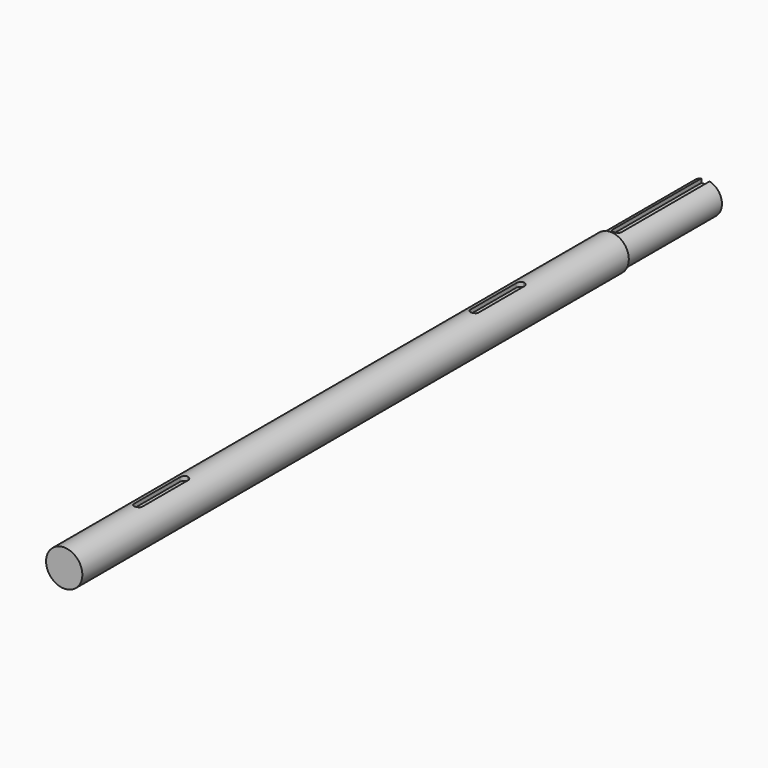
from build123d import *

# Parameters (mm, degrees)
F0_R      = 56.35625
F1_DEPTH  = 2120.9
F2_R      = 50.8
F3_DEPTH  = 368.3
F4_R      = 11.1125
F5_DEPTH  = 34.925
F6_W      = 25.4
F6_H      = 25.4
F7_DEPTH  = 355.6
F8_R      = 12.699
F11_DEPTH = 13.97


# Not quite as in the source:
# - a fillet or chamfer is up to 0.001 mm smaller than in the source, because OpenCascade refuses the exact size


with BuildPart() as f1:
    # F0 (on Front) → F1 (new body)
    with BuildSketch(Plane.XZ):
        Circle(F0_R)
    extrude(amount=-F1_DEPTH)

    # F2 (on face) → F3 (join)
    with BuildSketch(Plane(origin=(0, 2120.9, 0), x_dir=(-1, 0, 0), z_dir=(0, 1, 0))):
        Circle(F2_R)
    extrude(amount=F3_DEPTH)

    # F4 (on face) → F5 (cut)
    with BuildSketch(Plane(origin=(0, 2489.2, 0), x_dir=(-1, 0, 0), z_dir=(0, 1, 0))):
        Circle(F4_R)
    extrude(amount=-F5_DEPTH, mode=Mode.SUBTRACT)

    # F6 (on face) → F7 (cut)
    with BuildSketch(Plane(origin=(0, 2489.2, 0), x_dir=(-1, 0, 0), z_dir=(0, 1, 0))):
        with Locations((0, 49.53)):
            Rectangle(F6_W, F6_H)
    extrude(amount=-F7_DEPTH, mode=Mode.SUBTRACT)

    # F8 (radius 12.7 in the source; OpenCascade refuses exactly that, so slightly less here)
    f8_edges = [f1.edges().sort_by_distance(p)[0] for p in [
        (12.7, 2133.6, 43.008444),
        (-12.7, 2133.6, 43.008444),
    ]]
    fillet(f8_edges, radius=F8_R)

    # F10 (on offset) → F11 (cut)
    with BuildSketch(Plane.XY.offset(56.35625)):
        with BuildLine():
            ThreePointArc((0, 477.8375), (-8.9802561211, 474.1177561211), (-12.7, 465.1375))
            Line((-12.7, 465.1375), (-12.7, 287.3375))
            ThreePointArc((-12.7, 287.3375), (-8.9802561211, 278.3572438789), (0, 274.6375))
            ThreePointArc((0, 274.6375), (8.9802561211, 278.3572438789), (12.7, 287.3375))
            Line((12.7, 287.3375), (12.7, 465.1375))
            ThreePointArc((12.7, 465.1375), (8.9802561211, 474.1177561211), (0, 477.8375))
        make_face()
        with BuildLine():
            ThreePointArc((0, 1782.7625), (-8.9802561211, 1779.0427561211), (-12.7, 1770.0625))
            Line((-12.7, 1770.0625), (-12.7, 1592.2625))
            ThreePointArc((-12.7, 1592.2625), (-8.9802561211, 1583.2822438789), (0, 1579.5625))
            ThreePointArc((0, 1579.5625), (8.9802561211, 1583.2822438789), (12.7, 1592.2625))
            Line((12.7, 1592.2625), (12.7, 1770.0625))
            ThreePointArc((12.7, 1770.0625), (8.9802561211, 1779.0427561211), (0, 1782.7625))
        make_face()
    extrude(amount=-F11_DEPTH, mode=Mode.SUBTRACT)


solid = f1.part
